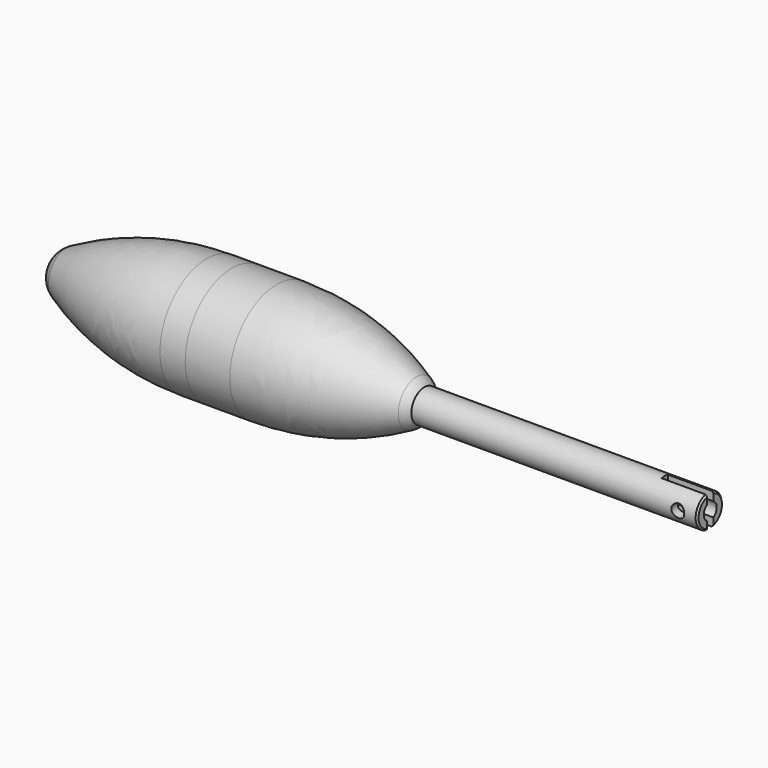
from build123d import *

# Parameters (mm, degrees)
F2_T      = -0.5
F3_SIZE   = 0.49999
F10_SIZE  = 0.25
F11_R     = 1
F12_DEPTH = 12.5
F13_W     = 1.2
F13_H     = 6
F14_DEPTH = 7


# Not quite as in the source:
# - a fillet or chamfer is up to 0.001 mm smaller than in the source, because OpenCascade refuses the exact size


with BuildPart() as f1:
    # F0 (on Front) → F1 (revolve)
    with BuildSketch(Plane.XZ):
        with BuildLine():
            Line((-30.5, 0), (0, 0))
            Line((0, 0), (0, 8.5))
            Line((0, 8.5), (-3, 8.5))
            Line((-3, 8.5), (-3, 9))
            Line((-3, 9), (-6.8785831297, 9))
            ThreePointArc((-6.8785831297, 9), (-17.990541092, 7.6064718848), (-28.4142845727, 3.512195122))
            ThreePointArc((-28.4142845727, 3.512195122), (-29.9392686934, 2.0424081019), (-30.5, 0))
        make_face()
    revolve(axis=Axis((-15.25, 0, 0), (1, 0, 0)))

    # F2
    f2_openings = [f1.faces().sort_by_distance(p)[0] for p in [
        (0, 0, 0),
    ]]
    offset(amount=F2_T, openings=f2_openings, kind=Kind.INTERSECTION)

    # F3 (size 0.5 in the source; OpenCascade refuses exactly that, so slightly less here)
    f3_edges = [f1.edges().sort_by_distance(p)[0] for p in [
        (-3.5, 0, -8),
    ]]
    chamfer(f3_edges, length=F3_SIZE)


with BuildPart() as f6:
    # F4 (on Front) → F6 (revolve)
    with BuildSketch(Plane.XZ):
        with BuildLine():
            Line((-3, 9), (-3, 0))
            Line((-3, 0), (26.62, 0))
            Line((26.62, 0), (26.62, 2.5048830838))
            ThreePointArc((26.62, 2.5048830838), (26.0677583739, 3.0682065261), (25.4157014431, 3.512195122))
            ThreePointArc((25.4157014431, 3.512195122), (14.9919579623, 7.6064718848), (3.88, 9))
            Line((3.88, 9), (-3, 9))
        make_face()
    revolve(axis=Axis((11.81, 0, 0), (-1, 0, 0)))

    # F5 (on Front) → F7 (revolve, cut)
    with BuildSketch(Plane.XZ):
        with BuildLine():
            Line((-3, 8.5), (-3, 0))
            Line((-3, 0), (26.62, 0))
            Line((26.62, 0), (26.62, 2))
            Line((26.62, 2), (20.623, 2))
            ThreePointArc((20.623, 2), (17.5537972972, 5.5481495418), (13.2852808385, 7.4947202813))
            ThreePointArc((13.2852808385, 7.4947202813), (8.6094263649, 8.2479663517), (3.88, 8.5))
            Line((3.88, 8.5), (-3, 8.5))
        make_face()
    revolve(axis=Axis((11.81, 0, 0), (-1, 0, 0)), mode=Mode.SUBTRACT)


with BuildPart() as f9:
    # F8 (on Front) → F9 (revolve)
    with BuildSketch(Plane.XZ):
        Polygon((20.62, 2), (20.62, 1.25), (70.62, 1.25), (70.62, 2.5), (26.62, 2.5), (26.62, 2), align=None)
    revolve(axis=Axis((45.62, 0, 0), (-1, 0, 0)))

    # F10
    f10_edges = [f9.edges().sort_by_distance(p)[0] for p in [
        (20.62, 0, -2),
        (70.62, 0, -2.5),
    ]]
    chamfer(f10_edges, length=F10_SIZE)

    # F11 (on Front) → F12 (cut, symmetric)
    with BuildSketch(Plane.XZ):
        with Locations((67.62, 0)):
            Circle(F11_R)
    extrude(amount=F12_DEPTH, both=True, mode=Mode.SUBTRACT)

    # F13 (on face) → F14 (cut)
    with BuildSketch(Plane.YZ.offset(70.62)):
        Rectangle(F13_W, F13_H)
    extrude(amount=-F14_DEPTH, mode=Mode.SUBTRACT)


solid = Compound([f1.part, f6.part, f9.part])
